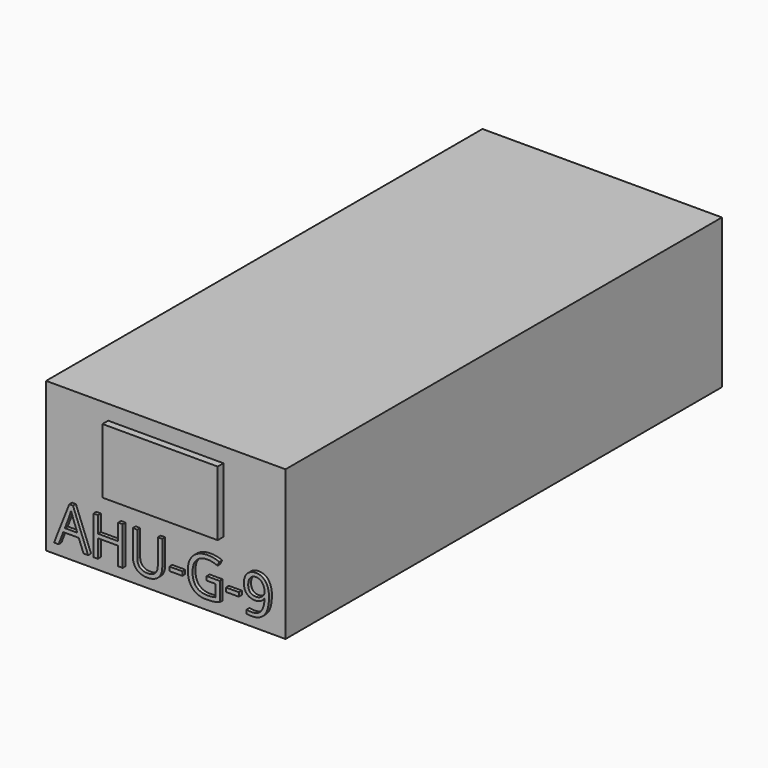
from build123d import *

# Parameters (mm, degrees)
F0_W         = 1689.1
F0_H         = 1054.1
F1_DEPTH     = 3848.1
F2_W         = 812.8
F2_H         = 457.2
F3_DEPTH     = 50.8
F4_TEXT_SIZE = 380.2978537149
F5_DEPTH     = 25.4
F6_W         = 1409.7
F6_H         = 431.8
F7_DEPTH     = 50.8
F8_W         = 1409.7
F8_H         = 431.8
F9_DEPTH     = 50.8


# Not quite as in the source:
# - Text() gives the source's letters only with a copy of the font that has no kerning and outlines rounded to 1/6400 em; it was checked with that copy


with BuildPart() as f1:
    # F0 (on Front) → F1 (new body)
    with BuildSketch(Plane.XZ):
        with Locations((204.6098696411, -25.3882179465)):
            Rectangle(F0_W, F0_H)
    extrude(amount=F1_DEPTH)

    # F2 (on face) → F3 (join)
    with BuildSketch(Plane.XZ.offset(3848.1)):
        with Locations((204.6098696411, 168.2867820535)):
            Rectangle(F2_W, F2_H)
    extrude(amount=F3_DEPTH)

    # F4 (on face) → F5 (join)
    with BuildSketch(Plane.XZ.offset(3848.1)):
        with Locations((-563.5762512684, -467.682570219)):
            Text('AHU-G-9', F4_TEXT_SIZE, font='Open Sans', text_align=(TextAlign.LEFT, TextAlign.BOTTOM))
    extrude(amount=F5_DEPTH)

    # F6 (on face) → F7 (join)
    with BuildSketch(Plane(origin=(0, 0, 0), x_dir=(-1, 0, 0), z_dir=(0, 1, 0))):
        with Locations((-204.6098696411, 9.5367820535)):
            Rectangle(F6_W, F6_H)
    extrude(amount=F7_DEPTH)

    # F8 (on face) → F9 (join)
    with BuildSketch(Plane(origin=(0, 0, -552.4382179465), x_dir=(1, 0, 0), z_dir=(0, 0, -1))):
        with Locations((204.6098696411, 282.575)):
            Rectangle(F8_W, F8_H)
    extrude(amount=F9_DEPTH)


solid = f1.part
